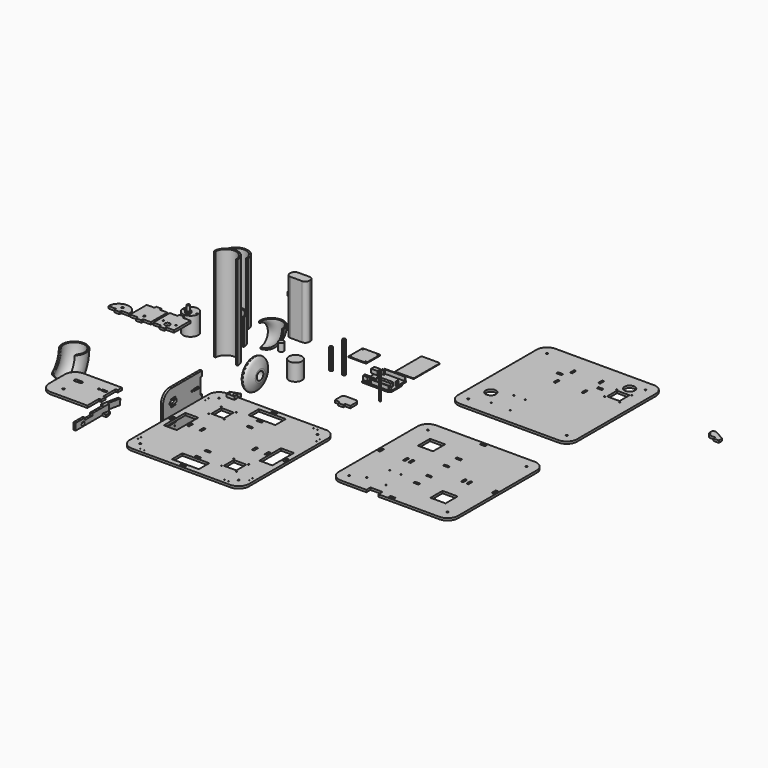
from build123d import *

# Parameters (mm, degrees)
F2_R      = 18.5
F2_R_2    = 6
F2_R_3    = 1.7
F2_R_4    = 3
F3_DEPTH  = 45.4
F4_R      = 6
F5_DEPTH  = 4
F6_R      = 3
F7_DEPTH  = 13
F8_W      = 43
F8_H      = 43
F8_R      = 1.7381100463
F9_DEPTH  = 2.032
F11_DEPTH = 132.08
F12_R     = 1.5875
F13_DEPTH = 3.175
F14_W     = 51.437207253
F14_H     = 1.8142834306
F14_W_2   = 43.0892407894
F14_H_2   = 1.5119016171
F14_W_3   = 35.6809198856
F14_H_3   = 7.1059428155
F14_R     = 2.2678673267
F14_R_2   = 2.4612020952
F14_W_4   = 12.0952129364
F14_H_4   = 6.349992007
F14_W_5   = 14.9678438902
F14_H_5   = 10.1297497749
F14_W_6   = 3.0238032341
F14_H_6   = 5.4428502917
F14_W_7   = 6.5011680126
F14_H_7   = 3.1749978662
F15_DEPTH = 9.525
F1_R      = 1.7
F1_R_2    = 6.25
F16_DEPTH = 5.4356
F1_R_3    = 2.4765
F17_R     = 2.1336
F17_R_2   = 1.016
F17_W     = 5.4356
F17_H     = 12.7
F17_W_2   = 31.75
F17_H_2   = 66.04
F17_W_3   = 5.0546
F17_W_4   = 12.7
F17_H_3   = 5.4356
F17_W_5   = 66.04
F17_H_4   = 31.75
F17_H_5   = 5.0546
F17_R_3   = 1.4605
F17_W_6   = 30.65
F17_H_6   = 30.65
F18_DEPTH = 5.4356
F20_DEPTH = 50.8
F21_DEPTH = 50.8
F22_DEPTH = 25.4
F24_R     = 2.1336
F24_R_2   = 1.5875
F24_W     = 5.4356
F24_H     = 12.7
F24_W_2   = 12.7
F24_H_2   = 5.4356
F24_W_3   = 36.9887980702
F24_H_3   = 36.9887980702
F24_H_4   = 5.0546
F24_W_4   = 5.0546
F25_DEPTH = 5.4356
F27_DEPTH = 5.4356
F29_R     = 29.21
F29_R_2   = 25.4
F30_ANGLE = 50
F31_W     = 38.1
F31_H     = 63.5
F32_DEPTH = 63.5
F33_R     = 1.2954
F33_R_2   = 0.889
F33_W     = 20.32
F33_H     = 8.382
F33_R_3   = 0.9016879686
F33_R_4   = 1.3
F33_R_5   = 2.1336
F33_W_2   = 12.7
F33_H_2   = 5.1816
F34_DEPTH = 5.4356
F35_R     = 2.5348881158
F35_R_2   = 2.1336
F35_W     = 12.7
F35_H     = 5.1816
F36_DEPTH = 5.4356
F28_R     = 2.1336
F28_R_2   = 1.5875
F28_R_3   = 12.7
F28_W     = 12.7
F28_H     = 5.4356
F28_W_2   = 5.0546
F28_H_2   = 12.7
F28_R_4   = 1.4605
F28_W_3   = 30.65
F28_H_3   = 30.65
F37_DEPTH = 5.4356
F39_DEPTH = 5.4356
F40_R     = 10.7315
F41_DEPTH = 5.4356
F43_ANGLE = 86
F45_DEPTH = 152.4
F47_DEPTH = 63.5
F49_DEPTH = 228.6
F50_R     = 16.0866870998
F51_DEPTH = 41.275
F55_DEPTH = 1.5494
F56_R     = 1.5875
F57_DEPTH = 63.5
F58_R     = 1.5193593542
F58_R_2   = 1.5422621567
F59_DEPTH = 7.62
F60_R     = 4.6270343152
F61_DEPTH = 5.4356
F63_DEPTH = 5.4356
F65_DEPTH = 5.08
F66_R     = 6.35
F67_DEPTH = 19.05


# Not quite as in the source:
# - a variable given as a bare number and used for a length is read in inches; the dataset says mm whatever the document's units were
# - a feature names something its author has since deleted; it is built from what else it names


with BuildPart() as f3:
    # F2 (on Top) → F3 (new body)
    with BuildSketch(Plane.XY):
        with Locations((-200.155207634, 64.0144571662)):
            Circle(F2_R)
        with Locations((-200.155207634, 57.0144571662)):
            Circle(F2_R_2, mode=Mode.SUBTRACT)
        with Locations((-215.655207634, 64.0144571662)):
            Circle(F2_R_3, mode=Mode.SUBTRACT)
        with Locations((-184.655207634, 64.0144571662)):
            Circle(F2_R_3, mode=Mode.SUBTRACT)
        with Locations((-200.155207634, 57.0144571662)):
            Circle(F2_R_2)
        with Locations((-200.155207634, 57.0144571662)):
            Circle(F2_R_4, mode=Mode.SUBTRACT)
        with Locations((-200.155207634, 57.0144571662)):
            Circle(F2_R_4)
    extrude(amount=-F3_DEPTH)

    # F4 (on face) → F5 (join)
    with BuildSketch(Plane.XY):
        with Locations((-200.155207634, 57.0144571662)):
            Circle(F4_R)
    extrude(amount=F5_DEPTH)

    # F6 (on face) → F7 (join)
    with BuildSketch(Plane.XY.offset(4)):
        with Locations((-200.155207634, 57.0144571662)):
            Circle(F6_R)
    extrude(amount=F7_DEPTH)


with BuildPart() as f9:
    # F8 (on Top) → F9 (new body)
    with BuildSketch(Plane.XY):
        with Locations((176.2737929821, 125.848295005)):
            Rectangle(F8_W, F8_H)
        with Locations((157.2153568268, 107.5413827896)):
            Circle(F8_R, mode=Mode.SUBTRACT)
        with Locations((194.2153568268, 107.5413827896)):
            Circle(F8_R, mode=Mode.SUBTRACT)
        with Locations((157.2153568268, 144.5413827896)):
            Circle(F8_R, mode=Mode.SUBTRACT)
        with Locations((194.2153568268, 144.5413827896)):
            Circle(F8_R, mode=Mode.SUBTRACT)
    extrude(amount=F9_DEPTH)


with BuildPart() as f11:
    # F10 (on Top) → F11 (new body)
    with BuildSketch(Plane.XY):
        with BuildLine():
            ThreePointArc((8.156953711, 107.2996626925), (11.1327488142, 100.1154577957), (18.316953711, 97.1396626925))
            Line((18.316953711, 97.1396626925), (46.256953711, 97.1396626925))
            ThreePointArc((46.256953711, 97.1396626925), (53.4411586079, 100.1154577957), (56.416953711, 107.2996626925))
            Line((56.416953711, 107.2996626925), (56.416953711, 109.8396626925))
            ThreePointArc((56.416953711, 109.8396626925), (53.4411586079, 117.0238675894), (46.256953711, 119.9996626925))
            Line((46.256953711, 119.9996626925), (18.316953711, 119.9996626925))
            ThreePointArc((18.316953711, 119.9996626925), (11.1327488142, 117.0238675894), (8.156953711, 109.8396626925))
            Line((8.156953711, 109.8396626925), (8.156953711, 107.2996626925))
        make_face()
    extrude(amount=F11_DEPTH)


with BuildPart() as f13:
    # F12 (on Top) → F13 (new body)
    with BuildSketch(Plane.XY):
        Polygon((305.0717792821, 92.5519884487), (240.3017792821, 92.5519884487), (240.3017792821, 38.5769884487), (305.0717792821, 38.5769884487), (305.0717792821, 40.9046933055), (308.9702129364, 43.6133395768), (308.9702129364, 75.2248838544), (305.0717792821, 78.551068902), align=None)
        with Locations((254.2717792821, 41.1169884487)):
            Circle(F12_R, mode=Mode.SUBTRACT)
        with Locations((306.3417792821, 46.1969884487)):
            Circle(F12_R, mode=Mode.SUBTRACT)
        with Locations((255.5417792821, 89.3769884487)):
            Circle(F12_R, mode=Mode.SUBTRACT)
        with Locations((306.3417792821, 74.1369884487)):
            Circle(F12_R, mode=Mode.SUBTRACT)
    extrude(amount=F13_DEPTH)

    # F14 (on face) → F15 (join)
    with BuildSketch(Plane.XY.offset(3.175)):
        with Locations((279.3531756556, 90.4950983822)):
            Rectangle(F14_W, F14_H)
        with Locations((282.2851389647, 40.602311492)):
            Rectangle(F14_W_2, F14_H_2)
        with Locations((282.814309001, 54.5874070376)):
            Rectangle(F14_W_3, F14_H_3)
        with Locations((255.9024393559, 46.6499216855)):
            Circle(F14_R)
        with Locations((261.1941099167, 46.6499216855)):
            Circle(F14_R_2)
        with Locations((244.5631623268, 46.3475417346)):
            Rectangle(F14_W_4, F14_H_4)
        with Locations((240.8590093255, 80.2897587419)):
            Rectangle(F14_W_5, F14_H_5)
        with Locations((304.2833209038, 66.0022757947)):
            Rectangle(F14_W_6, F14_H_6)
        with Locations((254.1637569666, 86.0349871218)):
            Rectangle(F14_W_7, F14_H_7)
    extrude(amount=F15_DEPTH)


with BuildPart() as f16:
    # F1 (on Top) → F16 (new body)
    with BuildSketch(Plane.XY):
        Polygon((-220.3947752714, 25.7545169817), (-220.3947752714, -25.0454830183), (-201.3447752714, -25.0454830183), (-201.3447752714, -30.4810830183), (-188.6447752714, -30.4810830183), (-188.6447752714, -25.0454830183), (-169.5947752714, -25.0454830183), (-169.5947752714, 25.7545169817), (-188.6447752714, 25.7545169817), (-188.6447752714, 31.1901169817), (-201.3447752714, 31.1901169817), (-201.3447752714, 25.7545169817), align=None)
        with Locations((-210.4947752714, -6.5454830183)):
            Circle(F1_R, mode=Mode.SUBTRACT)
        with Locations((-194.9947752714, -13.5454830183)):
            Circle(F1_R_2, mode=Mode.SUBTRACT)
        with Locations((-179.4947752714, -6.5454830183)):
            Circle(F1_R, mode=Mode.SUBTRACT)
    extrude(amount=F16_DEPTH)


with BuildPart() as f16b:
    # F1 (on Top) → F16, piece 2 (new body)
    with BuildSketch(Plane.XY):
        Polygon((-225.1267091751, -26.4407154173), (-225.1267091751, 24.3592845827), (-244.1767091751, 24.3592845827), (-244.1767091751, 29.7948845827), (-256.8767091751, 29.7948845827), (-256.8767091751, 24.3592845827), (-275.9267091751, 24.3592845827), (-275.9267091751, -26.4407154173), (-256.8767091751, -26.4407154173), (-256.8767091751, -31.8763154173), (-244.1767091751, -31.8763154173), (-244.1767091751, -26.4407154173), align=None)
        with Locations((-250.5267091751, -14.9407154173)):
            Circle(F1_R_3, mode=Mode.SUBTRACT)
    extrude(amount=F16_DEPTH)


with BuildPart() as f16c:
    # F1 (on Top) → F16, piece 3 (new body)
    with BuildSketch(Plane.XY):
        with BuildLine():
            Line((-298.6317808628, -25.0454830183), (-279.5817808628, -25.0454830183))
            ThreePointArc((-279.5817808628, -25.0454830183), (-304.9817808628, 0.3545169817), (-330.3817808628, -25.0454830183))
            Line((-330.3817808628, -25.0454830183), (-311.3317808628, -25.0454830183))
            Line((-311.3317808628, -25.0454830183), (-311.3317808628, -30.4810830183))
            Line((-311.3317808628, -30.4810830183), (-298.6317808628, -30.4810830183))
            Line((-298.6317808628, -30.4810830183), (-298.6317808628, -25.0454830183))
        make_face()
        with Locations((-304.9817808628, -13.5454830183)):
            Circle(F1_R_3, mode=Mode.SUBTRACT)
    extrude(amount=F16_DEPTH)


with BuildPart() as f18:
    # F17 (on Top) → F18 (new body)
    with BuildSketch(Plane.XY):
        with BuildLine():
            ThreePointArc((340.3421331108, -191.2749107361), (332.9026453529, -173.3143984939), (314.9421331108, -165.8749107361))
            Line((314.9421331108, -165.8749107361), (73.6421331108, -165.8749107361))
            ThreePointArc((73.6421331108, -165.8749107361), (55.6816208686, -173.3143984939), (48.2421331108, -191.2749107361))
            Line((48.2421331108, -191.2749107361), (48.2421331108, -432.5749107361))
            ThreePointArc((48.2421331108, -432.5749107361), (55.6816208686, -450.5354229782), (73.6421331108, -457.9749107361))
            Line((73.6421331108, -457.9749107361), (314.9421331108, -457.9749107361))
            ThreePointArc((314.9421331108, -457.9749107361), (332.9026453529, -450.5354229782), (340.3421331108, -432.5749107361))
            Line((340.3421331108, -432.5749107361), (340.3421331108, -191.2749107361))
        make_face()
        with Locations((73.6421331108, -432.5749107361)):
            Circle(F17_R, mode=Mode.SUBTRACT)
        with Locations((86.3421331108, -448.4499107361)):
            Circle(F17_R_2, mode=Mode.SUBTRACT)
        with Locations((95.8671331108, -448.4499107361)):
            Circle(F17_R_2, mode=Mode.SUBTRACT)
        with Locations((57.7671331108, -419.8749107361)):
            Circle(F17_R_2, mode=Mode.SUBTRACT)
        with Locations((57.7671331108, -410.3499107361)):
            Circle(F17_R_2, mode=Mode.SUBTRACT)
        with Locations((54.7699331108, -311.9249107361)):
            Rectangle(F17_W, F17_H, mode=Mode.SUBTRACT)
        with Locations((77.1727331108, -311.9249107361)):
            Rectangle(F17_W_2, F17_H_2, mode=Mode.SUBTRACT)
        with Locations((99.3850331108, -311.9249107361)):
            Rectangle(F17_W_3, F17_H, mode=Mode.SUBTRACT)
        with Locations((130.0301331108, -311.9249107361)):
            Rectangle(F17_W, F17_H, mode=Mode.SUBTRACT)
        with Locations((194.2921331108, -451.4471107361)):
            Rectangle(F17_W_4, F17_H_3, mode=Mode.SUBTRACT)
        with Locations((194.2921331108, -429.0443107361)):
            Rectangle(F17_W_5, F17_H_4, mode=Mode.SUBTRACT)
        with Locations((194.2921331108, -406.8320107361)):
            Rectangle(F17_W_4, F17_H_5, mode=Mode.SUBTRACT)
        with Locations((252.5421331108, -407.1749107361)):
            Circle(F17_R_3, mode=Mode.SUBTRACT)
        with Locations((292.7171331108, -448.4499107361)):
            Circle(F17_R_2, mode=Mode.SUBTRACT)
        with Locations((302.2421331108, -448.4499107361)):
            Circle(F17_R_2, mode=Mode.SUBTRACT)
        with Locations((314.9421331108, -432.5749107361)):
            Circle(F17_R, mode=Mode.SUBTRACT)
        with Locations((289.5421331108, -407.1749107361)):
            Circle(F17_R_3, mode=Mode.SUBTRACT)
        with Locations((271.0421331108, -388.6749107361)):
            Rectangle(F17_W_6, F17_H_6, mode=Mode.SUBTRACT)
        with Locations((330.8171331108, -419.8749107361)):
            Circle(F17_R_2, mode=Mode.SUBTRACT)
        with Locations((330.8171331108, -410.3499107361)):
            Circle(F17_R_2, mode=Mode.SUBTRACT)
        with Locations((194.2921331108, -376.1869107361)):
            Rectangle(F17_W_4, F17_H_3, mode=Mode.SUBTRACT)
        with Locations((252.5421331108, -370.1749107361)):
            Circle(F17_R_3, mode=Mode.SUBTRACT)
        with Locations((289.5421331108, -370.1749107361)):
            Circle(F17_R_3, mode=Mode.SUBTRACT)
        with Locations((99.0421331108, -253.6749107361)):
            Circle(F17_R_3, mode=Mode.SUBTRACT)
        with Locations((136.0421331108, -253.6749107361)):
            Circle(F17_R_3, mode=Mode.SUBTRACT)
        with Locations((57.7671331108, -213.4999107361)):
            Circle(F17_R_2, mode=Mode.SUBTRACT)
        with Locations((57.7671331108, -203.9749107361)):
            Circle(F17_R_2, mode=Mode.SUBTRACT)
        with Locations((117.5421331108, -235.1749107361)):
            Rectangle(F17_W_6, F17_H_6, mode=Mode.SUBTRACT)
        with Locations((99.0421331108, -216.6749107361)):
            Circle(F17_R_3, mode=Mode.SUBTRACT)
        with Locations((73.6421331108, -191.2749107361)):
            Circle(F17_R, mode=Mode.SUBTRACT)
        with Locations((86.3421331108, -175.3999107361)):
            Circle(F17_R_2, mode=Mode.SUBTRACT)
        with Locations((95.8671331108, -175.3999107361)):
            Circle(F17_R_2, mode=Mode.SUBTRACT)
        with Locations((136.0421331108, -216.6749107361)):
            Circle(F17_R_3, mode=Mode.SUBTRACT)
        with Locations((194.2921331108, -217.0178107361)):
            Rectangle(F17_W_4, F17_H_5, mode=Mode.SUBTRACT)
        with Locations((194.2921331108, -194.8055107361)):
            Rectangle(F17_W_5, F17_H_4, mode=Mode.SUBTRACT)
        with Locations((258.5541331108, -311.9249107361)):
            Rectangle(F17_W, F17_H, mode=Mode.SUBTRACT)
        with Locations((194.2921331108, -247.6629107361)):
            Rectangle(F17_W_4, F17_H_3, mode=Mode.SUBTRACT)
        with Locations((289.1992331108, -311.9249107361)):
            Rectangle(F17_W_3, F17_H, mode=Mode.SUBTRACT)
        with Locations((311.4115331108, -311.9249107361)):
            Rectangle(F17_W_2, F17_H_2, mode=Mode.SUBTRACT)
        with Locations((333.8143331108, -311.9249107361)):
            Rectangle(F17_W, F17_H, mode=Mode.SUBTRACT)
        with Locations((194.2921331108, -172.4027107361)):
            Rectangle(F17_W_4, F17_H_3, mode=Mode.SUBTRACT)
        with Locations((330.8171331108, -213.4999107361)):
            Circle(F17_R_2, mode=Mode.SUBTRACT)
        with Locations((330.8171331108, -203.9749107361)):
            Circle(F17_R_2, mode=Mode.SUBTRACT)
        with Locations((292.7171331108, -175.3999107361)):
            Circle(F17_R_2, mode=Mode.SUBTRACT)
        with Locations((302.2421331108, -175.3999107361)):
            Circle(F17_R_2, mode=Mode.SUBTRACT)
        with Locations((314.9421331108, -191.2749107361)):
            Circle(F17_R, mode=Mode.SUBTRACT)
    extrude(amount=F18_DEPTH)


with BuildPart() as f20:
    # F19 (on Top) → F20 (new body)
    with BuildSketch(Plane.XY):
        Polygon((166.3865149938, 41.3990794468), (164.3678937318, 44.8161168717), (160.3993418852, 44.7764582907), (158.4494113005, 41.3197622848), (160.4680325625, 37.9027248598), (164.4365844091, 37.9423834409), align=None)
    extrude(amount=F20_DEPTH)


with BuildPart() as f21:
    # F19 (on Top) → F21 (new body)
    with BuildSketch(Plane.XY):
        Polygon((166.3865149938, 41.3990794468), (164.3678937318, 44.8161168717), (160.3993418852, 44.7764582907), (158.4494113005, 41.3197622848), (160.4680325625, 37.9027248598), (164.4365844091, 37.9423834409), align=None)
    extrude(amount=F21_DEPTH)


with BuildPart() as f21b:
    # F19 (on Top) → F21, piece 2 (new body)
    with BuildSketch(Plane.XY):
        Polygon((196.9041229211, 42.7298015702), (194.8855016592, 46.1468389951), (190.9169498125, 46.1071804141), (188.9670192278, 42.6504844081), (190.9856404898, 39.2334469832), (194.9541923364, 39.2731055642), align=None)
    extrude(amount=F21_DEPTH)

    # F22 (add): a face of the model
    f22_faces = [f21b.faces().sort_by_distance(p)[0] for p in [
        (192.9355710745, 42.6901429892, 50.8),
    ]]
    extrude(f22_faces, amount=F22_DEPTH)


with BuildPart() as f25:
    # F24 (on Top) → F25 (new body)
    with BuildSketch(Plane.XY):
        with BuildLine():
            ThreePointArc((735.1522576593, -44.7709248373), (727.7127699014, -26.8104125951), (709.7522576593, -19.3709248373))
            Line((709.7522576593, -19.3709248373), (468.4522576593, -19.3709248373))
            ThreePointArc((468.4522576593, -19.3709248373), (450.4917454172, -26.8104125951), (443.0522576593, -44.7709248373))
            Line((443.0522576593, -44.7709248373), (443.0522576593, -286.0709248373))
            ThreePointArc((443.0522576593, -286.0709248373), (450.4917454172, -304.0314370794), (468.4522576593, -311.4709248373))
            Line((468.4522576593, -311.4709248373), (530.9023857117, -311.4709248373))
            Line((530.9023857117, -311.4709248373), (530.9023857117, -298.9526093006))
            Line((530.9023857117, -298.9526093006), (560.3792667389, -298.9526093006))
            Line((560.3792667389, -298.9526093006), (560.3792667389, -311.4709248373))
            Line((560.3792667389, -311.4709248373), (709.7522576593, -311.4709248373))
            ThreePointArc((709.7522576593, -311.4709248373), (727.7127699014, -304.0314370794), (735.1522576593, -286.0709248373))
            Line((735.1522576593, -286.0709248373), (735.1522576593, -44.7709248373))
        make_face()
        with Locations((468.4522576593, -286.0709248373)):
            Circle(F24_R, mode=Mode.SUBTRACT)
        with Locations((499.7121350288, -271.1671726799)):
            Circle(F24_R_2, mode=Mode.SUBTRACT)
        with Locations((547.9721350288, -272.4371726799)):
            Circle(F24_R_2, mode=Mode.SUBTRACT)
        with Locations((514.9521350288, -220.3671726799)):
            Circle(F24_R_2, mode=Mode.SUBTRACT)
        with Locations((449.5800576593, -165.4209248373)):
            Rectangle(F24_W, F24_H, mode=Mode.SUBTRACT)
        with Locations((542.8921350288, -220.3671726799)):
            Circle(F24_R_2, mode=Mode.SUBTRACT)
        with Locations((589.1022576593, -229.6829248373)):
            Rectangle(F24_W_2, F24_H_2, mode=Mode.SUBTRACT)
        with Locations((589.1022576593, -304.9431248373)):
            Rectangle(F24_W_2, F24_H_2, mode=Mode.SUBTRACT)
        with Locations((709.7522576593, -286.0709248373)):
            Circle(F24_R, mode=Mode.SUBTRACT)
        with Locations((665.8578586242, -242.1765258022)):
            Rectangle(F24_W_3, F24_H_3, mode=Mode.SUBTRACT)
        with Locations((589.1022576593, -192.0782248373)):
            Rectangle(F24_W_2, F24_H_4, mode=Mode.SUBTRACT)
        with Locations((511.6449576593, -165.4209248373)):
            Rectangle(F24_W_4, F24_H, mode=Mode.SUBTRACT)
        with Locations((524.8402576593, -165.4209248373)):
            Rectangle(F24_W, F24_H, mode=Mode.SUBTRACT)
        with Locations((589.1022576593, -138.7636248373)):
            Rectangle(F24_W_2, F24_H_4, mode=Mode.SUBTRACT)
        with Locations((512.3466566944, -88.6653238723)):
            Rectangle(F24_W_3, F24_H_3, mode=Mode.SUBTRACT)
        with Locations((468.4522576593, -44.7709248373)):
            Circle(F24_R, mode=Mode.SUBTRACT)
        with Locations((589.1022576593, -25.8987248373)):
            Rectangle(F24_W_2, F24_H_2, mode=Mode.SUBTRACT)
        with Locations((653.3642576593, -165.4209248373)):
            Rectangle(F24_W, F24_H, mode=Mode.SUBTRACT)
        with Locations((589.1022576593, -101.1589248373)):
            Rectangle(F24_W_2, F24_H_2, mode=Mode.SUBTRACT)
        with Locations((666.5595576593, -165.4209248373)):
            Rectangle(F24_W_4, F24_H, mode=Mode.SUBTRACT)
        with Locations((728.6244576593, -165.4209248373)):
            Rectangle(F24_W, F24_H, mode=Mode.SUBTRACT)
        with Locations((709.7522576593, -44.7709248373)):
            Circle(F24_R, mode=Mode.SUBTRACT)
    extrude(amount=F25_DEPTH)


with BuildPart() as f27:
    # F26 (on Top) → F27 (new body)
    with BuildSketch(Plane.XY):
        with BuildLine():
            ThreePointArc((289.5757155714, -39.8918483681), (287.7158436319, -35.4017203075), (283.2257155714, -33.5418483681))
            Line((283.2257155714, -33.5418483681), (257.8257155714, -33.5418483681))
            ThreePointArc((257.8257155714, -33.5418483681), (253.3355875109, -35.4017203075), (251.4757155714, -39.8918483681))
            Line((251.4757155714, -39.8918483681), (251.4757155714, -58.9418483681))
            Line((251.4757155714, -58.9418483681), (264.1757155714, -58.9418483681))
            Line((264.1757155714, -58.9418483681), (264.1757155714, -64.3774483681))
            Line((264.1757155714, -64.3774483681), (276.8757155714, -64.3774483681))
            Line((276.8757155714, -64.3774483681), (276.8757155714, -58.9418483681))
            Line((276.8757155714, -58.9418483681), (289.5757155714, -58.9418483681))
            Line((289.5757155714, -58.9418483681), (289.5757155714, -39.8918483681))
        make_face()
    extrude(amount=F27_DEPTH)


with BuildPart() as f30:
    # F29 (on Top) → F30 (revolve)
    with BuildSketch(Plane.XY):
        with Locations((-278.2541811466, -195.1718116283)):
            Circle(F29_R)
        with Locations((-278.2541811466, -195.1718116283)):
            Circle(F29_R_2, mode=Mode.SUBTRACT)
    revolve(axis=Axis((-297.1371263266, -271.3718116283, 0), (-1, 0, 0)), revolution_arc=F30_ANGLE)

    # F31 (on face) → F32 (cut)
    with BuildSketch(Plane.XY):
        with Locations((-278.2541811466, -242.1618116283)):
            Rectangle(F31_W, F31_H)
    extrude(amount=-F32_DEPTH, mode=Mode.SUBTRACT)


with BuildPart() as f34:
    # F33 (on Right) → F34 (new body)
    with BuildSketch(Plane.YZ):
        with BuildLine():
            Line((-157.4501020617, 29.2735), (-162.8857020617, 29.2735))
            Line((-162.8857020617, 29.2735), (-251.7857020617, 29.2735))
            ThreePointArc((-251.7857020617, 29.2735), (-269.7462143038, 21.8340122421), (-277.1857020617, 3.8735))
            Line((-277.1857020617, 3.8735), (-277.1857020617, -8.8265))
            Line((-277.1857020617, -8.8265), (-277.1857020617, -44.8818))
            ThreePointArc((-277.1857020617, -44.8818), (-269.7462143038, -62.8423122421), (-251.7857020617, -70.2818))
            Line((-251.7857020617, -70.2818), (-162.8857020617, -70.2818))
            Line((-162.8857020617, -70.2818), (-162.8857020617, -34.2265))
            Line((-162.8857020617, -34.2265), (-157.4501020617, -34.2265))
            Line((-157.4501020617, -34.2265), (-157.4501020617, -21.5265))
            Line((-157.4501020617, -21.5265), (-162.8857020617, -21.5265))
            Line((-162.8857020617, -21.5265), (-162.8857020617, 16.5735))
            Line((-162.8857020617, 16.5735), (-157.4501020617, 16.5735))
            Line((-157.4501020617, 16.5735), (-157.4501020617, 29.2735))
        make_face()
        with Locations((-241.6257020617, -55.6768)):
            Circle(F33_R, mode=Mode.SUBTRACT)
        with Locations((-259.4057020617, -44.8818)):
            Circle(F33_R_2, mode=Mode.SUBTRACT)
        with Locations((-247.9757020617, -44.8818)):
            Rectangle(F33_W, F33_H, mode=Mode.SUBTRACT)
        with Locations((-236.5457020617, -44.8818)):
            Circle(F33_R_3, mode=Mode.SUBTRACT)
        with Locations((-241.6257020617, -34.0868)):
            Circle(F33_R, mode=Mode.SUBTRACT)
        with Locations((-252.3557020617, -10.5908)):
            Circle(F33_R_4, mode=Mode.SUBTRACT)
        with Locations((-249.3557020617, -10.5908)):
            Circle(F33_R_4, mode=Mode.SUBTRACT)
        with Locations((-246.3557020617, -10.5908)):
            Circle(F33_R_4, mode=Mode.SUBTRACT)
        with Locations((-243.3557020617, -10.5908)):
            Circle(F33_R_4, mode=Mode.SUBTRACT)
        with Locations((-240.3557020617, -10.5908)):
            Circle(F33_R_4, mode=Mode.SUBTRACT)
        with BuildLine():
            Line((-252.3557020617, 2.4092), (-240.3557020617, 2.4092))
            ThreePointArc((-240.3557020617, 2.4092), (-236.8201681557, 0.9447339059), (-235.3557020617, -2.5908))
            ThreePointArc((-235.3557020617, -2.5908), (-236.8201681557, -6.1263339059), (-240.3557020617, -7.5908))
            Line((-240.3557020617, -7.5908), (-252.3557020617, -7.5908))
            ThreePointArc((-252.3557020617, -7.5908), (-255.8912359676, -6.1263339059), (-257.3557020617, -2.5908))
            ThreePointArc((-257.3557020617, -2.5908), (-255.8912359676, 0.9447339059), (-252.3557020617, 2.4092))
        make_face(mode=Mode.SUBTRACT)
        with Locations((-252.3557020617, 5.4092)):
            Circle(F33_R_4, mode=Mode.SUBTRACT)
        with Locations((-249.3557020617, 5.4092)):
            Circle(F33_R_4, mode=Mode.SUBTRACT)
        with Locations((-246.3557020617, 5.4092)):
            Circle(F33_R_4, mode=Mode.SUBTRACT)
        with Locations((-243.3557020617, 5.4092)):
            Circle(F33_R_4, mode=Mode.SUBTRACT)
        with Locations((-240.3557020617, 5.4092)):
            Circle(F33_R_4, mode=Mode.SUBTRACT)
        with Locations((-188.2857020617, -2.5908)):
            Circle(F33_R_5, mode=Mode.SUBTRACT)
        with Locations((-175.5857020617, -2.5908)):
            Rectangle(F33_W_2, F33_H_2, mode=Mode.SUBTRACT)
    extrude(amount=F34_DEPTH)


with BuildPart() as f36:
    # F35 (on Top) → F36 (new body)
    with BuildSketch(Plane.XY):
        with BuildLine():
            Line((-98.7353499653, -272.9478874207), (-104.1709499653, -272.9478874207))
            Line((-104.1709499653, -272.9478874207), (-193.0709499653, -272.9478874207))
            ThreePointArc((-193.0709499653, -272.9478874207), (-211.0314622075, -280.3873751785), (-218.4709499653, -298.3478874207))
            Line((-218.4709499653, -298.3478874207), (-218.4709499653, -311.0478874207))
            Line((-218.4709499653, -311.0478874207), (-218.4709499653, -346.8745874207))
            ThreePointArc((-218.4709499653, -346.8745874207), (-211.0314622075, -364.8350996628), (-193.0709499653, -372.2745874207))
            Line((-193.0709499653, -372.2745874207), (-104.1709499653, -372.2745874207))
            Line((-104.1709499653, -372.2745874207), (-104.1709499653, -336.4478874207))
            Line((-104.1709499653, -336.4478874207), (-98.7353499653, -336.4478874207))
            Line((-98.7353499653, -336.4478874207), (-98.7353499653, -323.7478874207))
            Line((-98.7353499653, -323.7478874207), (-104.1709499653, -323.7478874207))
            Line((-104.1709499653, -323.7478874207), (-104.1709499653, -285.6478874207))
            Line((-104.1709499653, -285.6478874207), (-98.7353499653, -285.6478874207))
            Line((-98.7353499653, -285.6478874207), (-98.7353499653, -272.9478874207))
        make_face()
        with Locations((-182.9109499653, -346.8745874207)):
            Circle(F35_R, mode=Mode.SUBTRACT)
        with BuildLine():
            ThreePointArc((-175.5209499653, -301.0812881759), (-170.2109499653, -304.5835874207), (-175.5209499653, -308.0858866654))
            ThreePointArc((-175.5209499653, -308.0858866654), (-177.0209499653, -308.3935874207), (-178.5209499653, -308.0858866654))
            ThreePointArc((-178.5209499653, -308.0858866654), (-180.0209499653, -308.3935874207), (-181.5209499653, -308.0858866654))
            ThreePointArc((-181.5209499653, -308.0858866654), (-183.0209499653, -308.3935874207), (-184.5209499653, -308.0858866654))
            ThreePointArc((-184.5209499653, -308.0858866654), (-189.8309499653, -304.5835874207), (-184.5209499653, -301.0812881759))
            ThreePointArc((-184.5209499653, -301.0812881759), (-183.0209499653, -300.7735874207), (-181.5209499653, -301.0812881759))
            ThreePointArc((-181.5209499653, -301.0812881759), (-180.0209499653, -300.7735874207), (-178.5209499653, -301.0812881759))
            ThreePointArc((-178.5209499653, -301.0812881759), (-177.0209499653, -300.7735874207), (-175.5209499653, -301.0812881759))
        make_face(mode=Mode.SUBTRACT)
        with Locations((-129.5709499653, -304.5835874207)):
            Circle(F35_R_2, mode=Mode.SUBTRACT)
        with Locations((-116.8709499653, -304.5835874207)):
            Rectangle(F35_W, F35_H, mode=Mode.SUBTRACT)
    extrude(amount=F36_DEPTH)


with BuildPart() as f37:
    # F28 (on Top) → F37 (new body)
    with BuildSketch(Plane.XY):
        with BuildLine():
            ThreePointArc((714.6546453957, 345.6536625793), (707.2151576378, 363.6141748215), (689.2546453957, 371.0536625793))
            Line((689.2546453957, 371.0536625793), (447.9546453957, 371.0536625793))
            ThreePointArc((447.9546453957, 371.0536625793), (429.9941331535, 363.6141748215), (422.5546453957, 345.6536625793))
            Line((422.5546453957, 345.6536625793), (422.5546453957, 104.3536625793))
            ThreePointArc((422.5546453957, 104.3536625793), (429.9941331535, 86.3931503372), (447.9546453957, 78.9536625793))
            Line((447.9546453957, 78.9536625793), (689.2546453957, 78.9536625793))
            ThreePointArc((689.2546453957, 78.9536625793), (707.2151576378, 86.3931503372), (714.6546453957, 104.3536625793))
            Line((714.6546453957, 104.3536625793), (714.6546453957, 345.6536625793))
        make_face()
        with Locations((447.9546453957, 104.3536625793)):
            Circle(F28_R, mode=Mode.SUBTRACT)
        with Locations((491.8088083618, 119.6018084884)):
            Circle(F28_R_2, mode=Mode.SUBTRACT)
        with Locations((540.0688083618, 118.3318084884)):
            Circle(F28_R_2, mode=Mode.SUBTRACT)
        with Locations((464.5873904228, 152.7419239283)):
            Circle(F28_R_3, mode=Mode.SUBTRACT)
        with Locations((507.0488083618, 170.4018084884)):
            Circle(F28_R_2, mode=Mode.SUBTRACT)
        with Locations((534.9888083618, 170.4018084884)):
            Circle(F28_R_2, mode=Mode.SUBTRACT)
        with Locations((689.2546453957, 104.3536625793)):
            Circle(F28_R, mode=Mode.SUBTRACT)
        with Locations((519.1000453957, 295.4886625793)):
            Rectangle(F28_W, F28_H, mode=Mode.SUBTRACT)
        with Locations((534.3273453957, 266.9136625793)):
            Rectangle(F28_W_2, F28_H_2, mode=Mode.SUBTRACT)
        with Locations((447.9546453957, 345.6536625793)):
            Circle(F28_R, mode=Mode.SUBTRACT)
        with Locations((534.3273453957, 317.7136625793)):
            Rectangle(F28_W_2, F28_H_2, mode=Mode.SUBTRACT)
        with Locations((602.8819453957, 266.9136625793)):
            Rectangle(F28_W_2, F28_H_2, mode=Mode.SUBTRACT)
        with Locations((618.1092453957, 295.4886625793)):
            Rectangle(F28_W, F28_H, mode=Mode.SUBTRACT)
        with Locations((645.5825567245, 275.218218565)):
            Circle(F28_R_4, mode=Mode.SUBTRACT)
        with Locations((664.0825567245, 293.718218565)):
            Rectangle(F28_W_3, F28_H_3, mode=Mode.SUBTRACT)
        with Locations((682.5825567245, 275.218218565)):
            Circle(F28_R_4, mode=Mode.SUBTRACT)
        with Locations((602.8819453957, 317.7136625793)):
            Rectangle(F28_W_2, F28_H_2, mode=Mode.SUBTRACT)
        with Locations((645.5825567245, 312.218218565)):
            Circle(F28_R_4, mode=Mode.SUBTRACT)
        with Locations((662.2430086136, 330.8306336403)):
            Circle(F28_R_3, mode=Mode.SUBTRACT)
        with Locations((682.5825567245, 312.218218565)):
            Circle(F28_R_4, mode=Mode.SUBTRACT)
        with Locations((689.2546453957, 345.6536625793)):
            Circle(F28_R, mode=Mode.SUBTRACT)
    extrude(amount=F37_DEPTH)


with BuildPart() as f39:
    # F38 (on Top) → F39 (new body)
    with BuildSketch(Plane.XY):
        with BuildLine():
            Line((902.1028009221, 294.1765774727), (901.0572369581, 294.1765774727))
            Line((901.0572369581, 294.1765774727), (895.6216369581, 294.1765774727))
            Line((895.6216369581, 294.1765774727), (895.6216369581, 281.4765774727))
            Line((895.6216369581, 281.4765774727), (901.0572369581, 281.4765774727))
            Line((901.0572369581, 281.4765774727), (901.0572369581, 275.1265774727))
            Line((901.0572369581, 275.1265774727), (916.9322369581, 275.1265774727))
            Line((916.9322369581, 275.1265774727), (916.9322369581, 269.6909774727))
            Line((916.9322369581, 269.6909774727), (929.6322369581, 269.6909774727))
            Line((929.6322369581, 269.6909774727), (929.6322369581, 275.1265774727))
            Line((929.6322369581, 275.1265774727), (929.6322369581, 278.1280651167))
            ThreePointArc((929.6322369581, 278.1280651167), (929.1882596255, 279.7473674943), (927.980495106, 280.9137983442))
            Line((927.980495106, 280.9137983442), (905.1493172178, 293.3980439278))
            ThreePointArc((905.1493172178, 293.3980439278), (903.6750108334, 293.9788661521), (902.1028009221, 294.1765774727))
        make_face()
    extrude(amount=F39_DEPTH)


with BuildPart() as f41:
    # F40 (on Top) → F41 (new body)
    with BuildSketch(Plane.XY):
        with Locations((-89.9502384677, 239.5131986534)):
            Circle(F40_R)
        with BuildLine():
            ThreePointArc((-88.0467630778, 241.8118986534), (-89.9502384677, 236.5286986534), (-91.8537138576, 241.8118986534))
            Line((-91.8537138576, 241.8118986534), (-88.0467630778, 241.8118986534))
        make_face(mode=Mode.SUBTRACT)
    extrude(amount=F41_DEPTH)


with BuildPart() as f43:
    # F42 (on Top) → F43 (revolve)
    with BuildSketch(Plane.XY):
        with BuildLine():
            ThreePointArc((-69.2484222893, 117.0122962834), (-43.849676476, 142.1598856807), (-18.4509306627, 117.0122962834))
            Line((-18.4509306627, 117.0122962834), (-14.6407670666, 117.0122962834))
            ThreePointArc((-14.6407670666, 117.0122962834), (-43.849676476, 145.9698856807), (-73.0585858854, 117.0122962834))
            Line((-73.0585858854, 117.0122962834), (-69.2484222893, 117.0122962834))
        make_face()
    revolve(axis=Axis((-75.599676476, 78.5722535253, 0), (0, 1, 0)), revolution_arc=F43_ANGLE)


with BuildPart() as f45:
    # F44 (on Top) → F45 (new body)
    with BuildSketch(Plane.XY):
        with BuildLine():
            ThreePointArc((-122.5255782985, 73.9049157609), (-97.1268324852, 99.0525051582), (-71.7280866719, 73.9049157609))
            Line((-71.7280866719, 73.9049157609), (-67.9179230758, 73.9049157609))
            ThreePointArc((-67.9179230758, 73.9049157609), (-97.1268324852, 102.8625051582), (-126.3357418946, 73.9049157609))
            Line((-126.3357418946, 73.9049157609), (-122.5255782985, 73.9049157609))
        make_face()
    extrude(amount=F45_DEPTH)


with BuildPart() as f47:
    # F46 (on Top) → F47 (new body)
    with BuildSketch(Plane.XY):
        with BuildLine():
            ThreePointArc((-82.8906576418, 12.1506061887), (-57.4919118285, 37.298195586), (-32.0931660152, 12.1506061887))
            Line((-32.0931660152, 12.1506061887), (-28.2830024191, 12.1506061887))
            ThreePointArc((-28.2830024191, 12.1506061887), (-57.4919118285, 41.108195586), (-86.7008212379, 12.1506061887))
            Line((-86.7008212379, 12.1506061887), (-82.8906576418, 12.1506061887))
        make_face()
    extrude(amount=F47_DEPTH)


with BuildPart() as f49:
    # F48 (on Top) → F49 (new body)
    with BuildSketch(Plane.XY):
        with BuildLine():
            ThreePointArc((-43.5696970009, -55.5982598553), (-18.1709511876, -30.450670458), (7.2277946257, -55.5982598553))
            Line((7.2277946257, -55.5982598553), (11.0379582218, -55.5982598553))
            ThreePointArc((11.0379582218, -55.5982598553), (-18.1709511876, -26.640670458), (-47.379860597, -55.5982598553))
            Line((-47.379860597, -55.5982598553), (-43.5696970009, -55.5982598553))
        make_face()
    extrude(amount=F49_DEPTH)


with BuildPart() as f51:
    # F50 (on Top) → F51 (new body)
    with BuildSketch(Plane.XY):
        with Locations((128.865301609, -26.0448567569)):
            Circle(F50_R)
    extrude(amount=F51_DEPTH)


with BuildPart() as f53:
    # F52 (on Top) → F53 (revolve)
    with BuildSketch(Plane.XY):
        with BuildLine():
            Line((45.1035822575, -51.4359772205), (70.5035822575, -51.4359772205))
            Line((70.5035822575, -51.4359772205), (70.5035822575, -46.5381145477))
            add(Edge.make_bspline(
                [(57.8035822575, -24.4616798174), (58.1046127752, -24.4828729684), (58.8309796715, -24.5340106518), (60.8619737919, -25.1828219157), (63.6062263354, -27.1159789027), (67.7573602064, -37.2672439221), (69.5960889334, -43.4745410112), (70.5035822575, -46.5381145477)],
                knots=[0, 0, 0, 0, 0.0936740846, 0.2260294226, 0.3927455367, 0.7002932715, 1, 1, 1, 1], degree=3))
            add(Edge.make_bspline(
                [(57.8035822575, -24.4616798174), (57.5025517398, -24.4828729684), (56.7761848435, -24.5340106518), (54.7451907231, -25.1828219157), (52.0009381796, -27.1159789027), (47.8498043086, -37.2672439221), (46.0110755816, -43.4745410112), (45.1035822575, -46.5381145477)],
                knots=[0, 0, 0, 0, 0.0936740846, 0.2260294226, 0.3927455367, 0.7002932715, 1, 1, 1, 1], degree=3))
            Line((45.1035822575, -46.5381145477), (45.1035822575, -51.4359772205))
        make_face()
    revolve(axis=Axis((57.8035822575, -61.4186798174, 0), (-1, 0, 0)))


with BuildPart() as f55:
    # F54 (on Top) → F55 (new body)
    with BuildSketch(Plane.XY):
        with BuildLine():
            Line((285.7218478775, 192.6153784657), (265.4018478775, 192.6153784657))
            ThreePointArc((265.4018478775, 192.6153784657), (263.6057966533, 191.8714296899), (262.8618478775, 190.0753784657))
            Line((262.8618478775, 190.0753784657), (262.8618478775, 113.8753784657))
            ThreePointArc((262.8618478775, 113.8753784657), (263.6057966533, 112.0793272414), (265.4018478775, 111.3353784657))
            Line((265.4018478775, 111.3353784657), (285.7218478775, 111.3353784657))
            Line((285.7218478775, 111.3353784657), (306.0418478775, 111.3353784657))
            ThreePointArc((306.0418478775, 111.3353784657), (307.8378991017, 112.0793272414), (308.5818478775, 113.8753784657))
            Line((308.5818478775, 113.8753784657), (308.5818478775, 190.0753784657))
            ThreePointArc((308.5818478775, 190.0753784657), (307.8378991017, 191.8714296899), (306.0418478775, 192.6153784657))
            Line((306.0418478775, 192.6153784657), (285.7218478775, 192.6153784657))
        make_face()
    extrude(amount=F55_DEPTH)


with BuildPart() as f57:
    # F56 (on Top) → F57 (new body)
    with BuildSketch(Plane.XY):
        with Locations((315.3353333473, 0)):
            Circle(F56_R)
    extrude(amount=F57_DEPTH)


with BuildPart() as f59:
    # F58 (on face) → F59 (new body)
    with BuildSketch(Plane.XY.offset(5.4356)):
        with BuildLine():
            Line((84.491610527, -168.3028191328), (82.0610001683, -168.3028191328))
            Line((82.0610001683, -168.3028191328), (82.0610001683, -178.4493029118))
            Line((82.0610001683, -178.4493029118), (100.8853912354, -178.4493029118))
            Line((100.8853912354, -178.4493029118), (100.8853912354, -168.3028191328))
            Line((100.8853912354, -168.3028191328), (86.496219039, -168.3028191328))
            Line((86.496219039, -168.3028191328), (101.7312135111, -163.6647482662))
            ThreePointArc((101.7312135111, -163.6647482662), (104.5842542331, -162.1797586869), (101.3990691965, -162.6265603145))
            Line((101.3990691965, -162.6265603145), (84.491610527, -168.3028191328))
        make_face()
        with Locations((86.3421331108, -175.3999107361)):
            Circle(F58_R, mode=Mode.SUBTRACT)
        with Locations((95.8671331108, -175.3999107361)):
            Circle(F58_R_2, mode=Mode.SUBTRACT)
    extrude(amount=F59_DEPTH)


with BuildPart() as f61:
    # F60 (on Right) → F61 (new body)
    with BuildSketch(Plane.YZ):
        Polygon((-544.9204444885, 56.9736920297), (-443.4724748135, 56.9736920297), (-443.4724748135, 73.52796942), (-494.196459651, 73.52796942), (-494.196459651, 68.4930309653), (-516.2650346756, 68.4930309653), (-516.2650346756, 73.52796942), (-544.9204444885, 73.52796942), align=None)
        with Locations((-522.0366120338, 62.7214834094)):
            Circle(F60_R, mode=Mode.SUBTRACT)
    extrude(amount=F61_DEPTH)

    # F62 (on face) → F63 (join)
    with BuildSketch(Plane(origin=(0, 0, 0), x_dir=(0, -1, 0), z_dir=(-1, 0, 0))):
        Polygon((403.0739846319, 52.3896192921), (455.3773721014, 59.7403810248), (453.4396529198, 73.52796942), (401.1362654503, 66.1772076872), align=None)
    extrude(amount=F63_DEPTH)


with BuildPart() as f65:
    # F64 (on face) → F65 (new body)
    with BuildSketch(Plane(origin=(0, -0.586933221, -4.1762468701), x_dir=(1, 0, 0), z_dir=(0, -0.139173101, -0.9902680687))):
        Polygon((14.0948632991, 465.9143808887), (-4.9551367009, 465.9143808887), (-4.9551367009, 459.5643808887), (0.7598632991, 446.8643808887), (8.3798632991, 446.8643808887), (14.0948632991, 459.5643808887), align=None)
    extrude(amount=F65_DEPTH)


with BuildPart() as f67:
    # F66 (on Top) → F67 (new body)
    with BuildSketch(Plane.XY):
        with Locations((36.483258009, 45.9861457348)):
            Circle(F66_R)
    extrude(amount=F67_DEPTH)


solid = Compound([f3.part, f9.part, f11.part, f13.part, f16.part, f16b.part, f16c.part, f18.part, f20.part, f21b.part, f25.part, f27.part, f30.part, f34.part, f36.part, f37.part, f39.part, f41.part, f43.part, f45.part, f47.part, f49.part, f51.part, f53.part, f55.part, f57.part, f59.part, f61.part, f65.part, f67.part])
